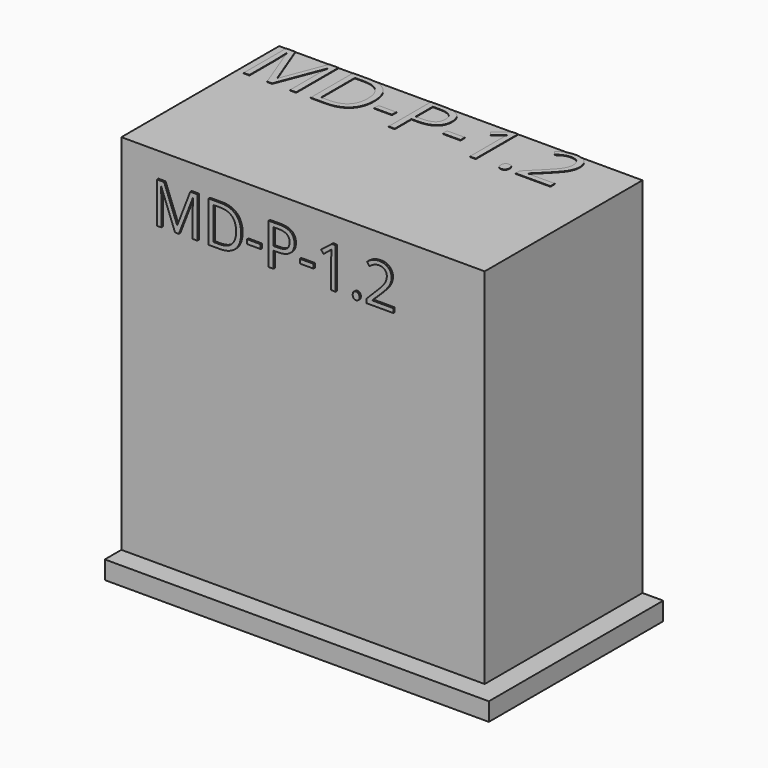
from build123d import *

# Parameters (mm, degrees)
F0_W         = 1778
F0_H         = 711.2
F1_DEPTH     = 1778
F2_TEXT_SIZE = 279.6484364404
F3_DEPTH     = 6.35
F4_DEPTH     = 254
F5_DEPTH     = 254
F6_DEPTH     = 256.54
F7_DEPTH     = 88.9
F8_TEXT_SIZE = 363.0090520779
F9_DEPTH     = 2.54
F10_W        = 1778
F10_H        = 88.9
F11_DEPTH    = 101.6
F13_DEPTH    = 101.6


# Not quite as in the source:
# - Text() gives the source's letters only with a copy of the font that has no kerning and outlines rounded to 1/6400 em; it was checked with that copy


with BuildPart() as f1:
    # F0 (on Top) → F1 (new body)
    with BuildSketch(Plane.XY):
        with Locations((889, 355.6)):
            Rectangle(F0_W, F0_H)
    extrude(amount=F1_DEPTH)

    # F2 (on face) → F3 (join)
    with BuildSketch(Plane.XZ):
        with Locations((153.9272218943, 1458.6802721024)):
            Text('MD-P-1.2', F2_TEXT_SIZE, font='Open Sans', text_align=(TextAlign.LEFT, TextAlign.BOTTOM))
    extrude(amount=F3_DEPTH)

    # F4 (add): a face of the model
    f4_faces = [f1.faces().sort_by_distance(p)[0] for p in [
        (895.0472022616, 0, 871.7793837697),
    ]]
    extrude(f4_faces, amount=F4_DEPTH)

    # F5 (add): faces of the model
    f5_faces = [f1.faces().sort_by_distance(p)[0] for p in [
        (507.3458158111, 0, 1558.8791853686),
        (786.9789876531, 0, 1597.8762050397),
    ]]
    extrude(f5_faces, amount=F5_DEPTH)

    # F6 (add): faces of the model
    f6_faces = [f1.faces().sort_by_distance(p)[0] for p in [
        (238.4796679926, -6.35, 1548.1671060625),
        (590.5899270597, -6.35, 1556.23546607),
        (851.8342710142, -6.35, 1596.647461151),
        (655.28443435, -6.35, 1533.6391615888),
        (913.6096775118, -6.35, 1533.6391615888),
        (1038.6640086696, -6.35, 1571.6545561316),
        (1155.5811793405, -6.35, 1473.2334316088),
        (1272.1495595761, -6.35, 1461.0930932367),
    ]]
    extrude(f6_faces, amount=F6_DEPTH)

    # F7 (add): a face of the model
    f7_faces = [f1.faces().sort_by_distance(p)[0] for p in [
        (889, 228.6, 0),
    ]]
    extrude(f7_faces, amount=F7_DEPTH)

    # F8 (on face) → F9 (join)
    with BuildSketch(Plane.XY.offset(1778)):
        with Locations((0, 449.8334825039)):
            Text('MD-P-1.2', F8_TEXT_SIZE, font='Open Sans', text_align=(TextAlign.LEFT, TextAlign.BOTTOM))
    extrude(amount=F9_DEPTH)

    # F10 (on face) → F11 (join)
    with BuildSketch(Plane.XZ.offset(254)):
        with Locations((889, -44.45)):
            Rectangle(F10_W, F10_H)
    extrude(amount=F11_DEPTH)

    # F12 (on face) → F13 (join)
    with BuildSketch(Plane.YZ.offset(1778)):
        Polygon((-355.6, 0), (-355.6, -88.9), (711.2, -88.9), (711.2, 0), (-254, 0), align=None)
    extrude(amount=F13_DEPTH)


solid = f1.part
